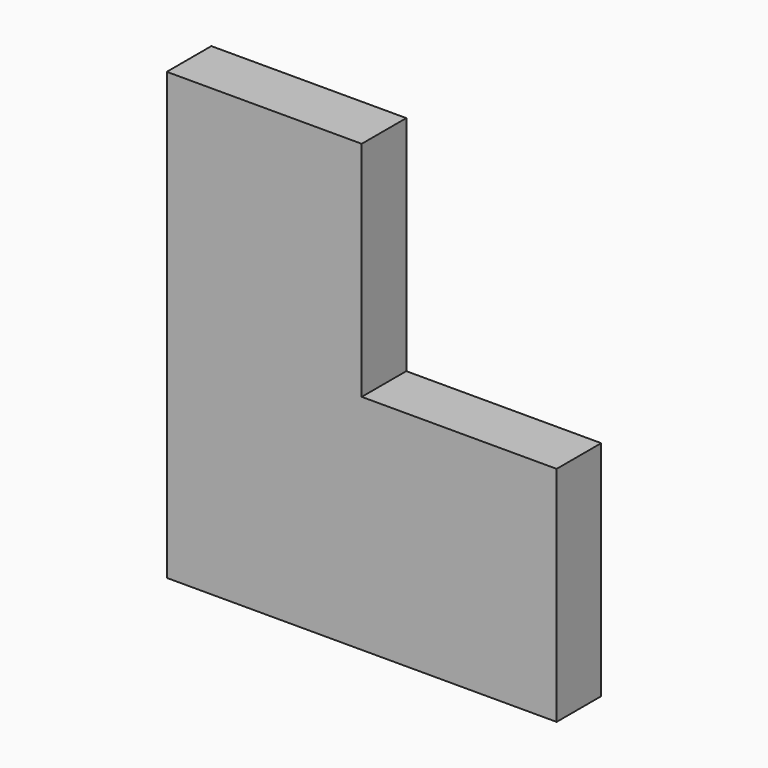
from build123d import *

# Parameters (mm, degrees)
F1_DEPTH = 12.7


# Not quite as in the source:
# - a length typed as a fraction of an inch, garbled in the dataset ("3 / 203.2 mm" for 3/8 in), is restored


with BuildPart() as f1:
    # F0 (on Front) → F1 (new body)
    with BuildSketch(Plane.XZ):
        Polygon((0, 101.6), (0, 0), (88.9, 0), (88.9, 50.8), (44.45, 50.8), (44.45, 101.6), align=None)
    extrude(amount=F1_DEPTH)


solid = f1.part
